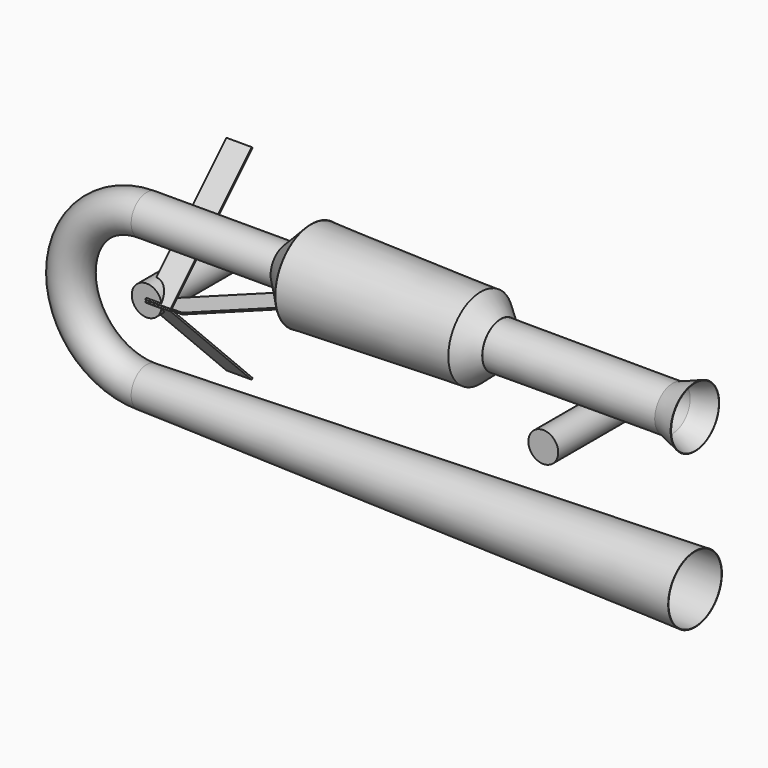
from build123d import *

# Parameters (mm, degrees)
F0_W        = 280
F0_H        = 0.9
F1_FACE_R   = 38.9
F1_FACE_R_2 = 38
F0_R        = 30
F4_DEPTH    = 203.2
F7_DEPTH    = 50.8
F10_DEPTH   = 1.5875


# Not quite as in the source:
# - a length typed as a fraction of an inch, garbled in the dataset ("3 / 203.2 mm" for 3/8 in), is restored


with BuildPart() as f1:
    # F0 (on Front) → F1 (revolve)
    with BuildSketch(Plane.XZ):
        Polygon((-0.3015087009, -60.8479932213), (0, -60), (-45, -44), (-45, -44.9551963149), align=None)
        Polygon((-45, -44.9551963149), (-45, -44), (-390, -45), (-390, -45.9551963149), align=None)
        Polygon((-390, -45.9551963149), (-390, -45), (-430, -80), (-430, -80.9003152562), (-430, -81.1958914039), (-390, -46.1958914039), align=None)
        Polygon((-430, -80.9003152562), (-430, -80), (-770, -89), (-770, -89.9003152562), align=None)
        Polygon((-770, -89.9003152562), (-770, -89), (-820, -38), (-820, -38.9), (-820, -39.2855831362), (-770, -90.2855831362), align=None)
        with Locations((-960, -38.45)):
            Rectangle(F0_W, F0_H)
    revolve(axis=Axis((-550, 0, 0), (-1, 0, 0)))

    # F2: sweep along a path in F0
    with BuildLine(Plane.XZ) as f2_path:
        ThreePointArc((-1100, -38.9), (-1213.1, -152), (-1100, -265.1))
    # F1_face (on face) → F2 (sweep)
    with BuildSketch(Plane(origin=(-1100, 0, 0), x_dir=(0, -1, 0), z_dir=(-1, 0, 0))):
        Circle(F1_FACE_R)
        Circle(F1_FACE_R_2, mode=Mode.SUBTRACT)
    sweep(path=f2_path.line)

    # F0 (on Front) → F3 (revolve)
    with BuildSketch(Plane.XZ):
        Polygon((-1100, -265.1), (-1100, -266), (0, -237.5), (0, -236.5996979742), (-1100, -265.0996979742), align=None)
    revolve(axis=Axis((-383.8686078787, 0, -304), (1, 0, 0)))


with BuildPart() as f4:
    # F0 (on Front) → F4 (new body)
    with BuildSketch(Plane.XZ):
        with Locations((-1100, -152)):
            Circle(F0_R)
    extrude(amount=-F4_DEPTH)


with BuildPart() as f4b:
    # F0 (on Front) → F4, piece 2 (new body)
    with BuildSketch(Plane.XZ):
        with Locations((-304.4275343418, -152)):
            Circle(F0_R)
    extrude(amount=-F4_DEPTH)


with BuildPart() as f7:
    # F6 (on offset) → F7 (new body)
    with BuildSketch(Plane.YZ.offset(-1101)):
        Polygon((-2.2450640303, -149.7549359697), (0, -152), (203.2, 51.2), (200.9549359697, 53.4450640303), align=None)
    extrude(amount=F7_DEPTH)


with BuildPart() as f7b:
    # F6 (on offset) → F7, piece 2 (new body)
    with BuildSketch(Plane.YZ.offset(-1101)):
        Polygon((203.2, -355.2), (0, -152), (-2.2450640303, -154.2450640303), (200.9549359697, -357.4450640303), align=None)
    extrude(amount=F7_DEPTH)


with BuildPart() as f10:
    # F9 (on offset) → F10 (new body, symmetric)
    with BuildSketch(Plane.XY.offset(-152)):
        Polygon((-1100, 0), (-1028.4874627811, 0), (-827.1557770688, 203.2), (-898.6683142877, 203.2), align=None)
    extrude(amount=F10_DEPTH, both=True)


solid = Compound([f1.part, f4.part, f4b.part, f7.part, f7b.part, f10.part])
